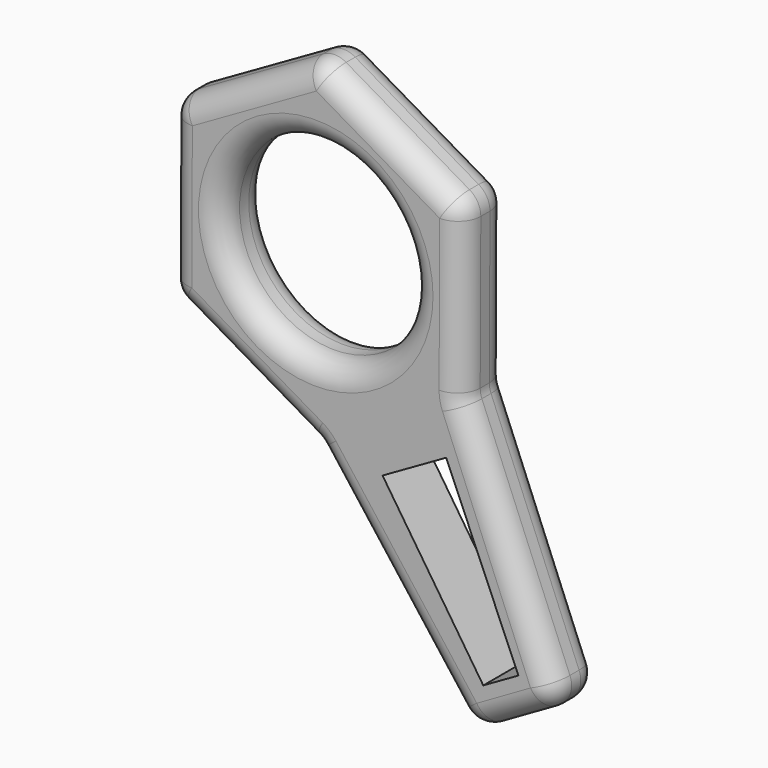
from build123d import *

# Parameters (mm, degrees)
F0_R     = 21.014231477
F1_DEPTH = 12.7
F2_F1_R  = 5.08
F2_F2_R  = 5.08


with BuildPart() as f1:
    # F0 (on Front) → F1 (new body)
    with BuildSketch(Plane.XZ):
        Polygon((-7.8242197393, -24.2327329676), (24.8512287471, -5.5456817597), (25.0054919224, 32.0956123135), (-7.5156933887, 51.0498551788), (-40.1911418751, 32.3628039709), (-40.3454050504, -5.2784901024), align=None)
        with Locations((-7.669956564, 13.4085611056)):
            Circle(F0_R, mode=Mode.SUBTRACT)
        Polygon((46.5040828879, -58.4152766954), (24.8512287471, -5.5456817597), (-7.8242197393, -24.2327329676), (26.8212909929, -69.7477493281), align=None)
        Polygon((29.6051679054, -59.1493866598), (7.1951453574, -25.3269076347), (21.3564252001, -17.2280880668), (37.4147482216, -54.6830967069), align=None, mode=Mode.SUBTRACT)
    extrude(amount=F1_DEPTH)

    # F2: fillet of radius 5.08 on 22 edges, made by hand

    # F2_f1
    f2_f1_edges = [f1.edges().sort_by_distance(p)[0] for p in [
        (-7.8242197393, -6.35, -24.2327329676),
        (24.8512287471, -6.35, -5.5456817597),
    ]]
    fillet(f2_f1_edges, radius=F2_F1_R)

    # F2_f2
    f2_f2_edges = [f1.edges().sort_by_distance(p)[0] for p in [
        (-28.684188041, -12.7, 13.4085611056),
        (-40.3454050504, -6.35, -5.2784901024),
        (-24.5210673055, 0, -14.5013501528),
        (-24.5210673055, -12.7, -14.5013501528),
        (-40.1911418751, -6.35, 32.3628039709),
        (-40.2682734628, 0, 13.5421569342),
        (-40.2682734628, -12.7, 13.5421569342),
        (26.8212909929, -6.35, -69.7477493281),
        (46.5040828879, -6.35, -58.4152766954),
        (36.6626869404, 0, -64.0815130117),
        (36.6626869404, -12.7, -64.0815130117),
        (35.8691964804, 0, -32.4481624806),
        (35.8691964804, -12.7, -32.4481624806),
        (25.0054919224, -6.35, 32.0956123135),
        (-7.5156933887, -6.35, 51.0498551788),
        (8.7448992668, 0, 41.5727337462),
        (8.7448992668, -12.7, 41.5727337462),
        (-23.8534176319, 0, 41.7063295748),
        (-23.8534176319, -12.7, 41.7063295748),
        (-28.684188041, 0, 13.4085611056),
        (24.9489742828, -12.7, -5.5266493336),
        (24.9489742828, 0, -5.5266493336),
        (-7.8900615225, -12.7, -24.3072100781),
        (-7.8900615225, 0, -24.3072100781),
    ]]
    fillet(f2_f2_edges, radius=F2_F2_R)


solid = f1.part
